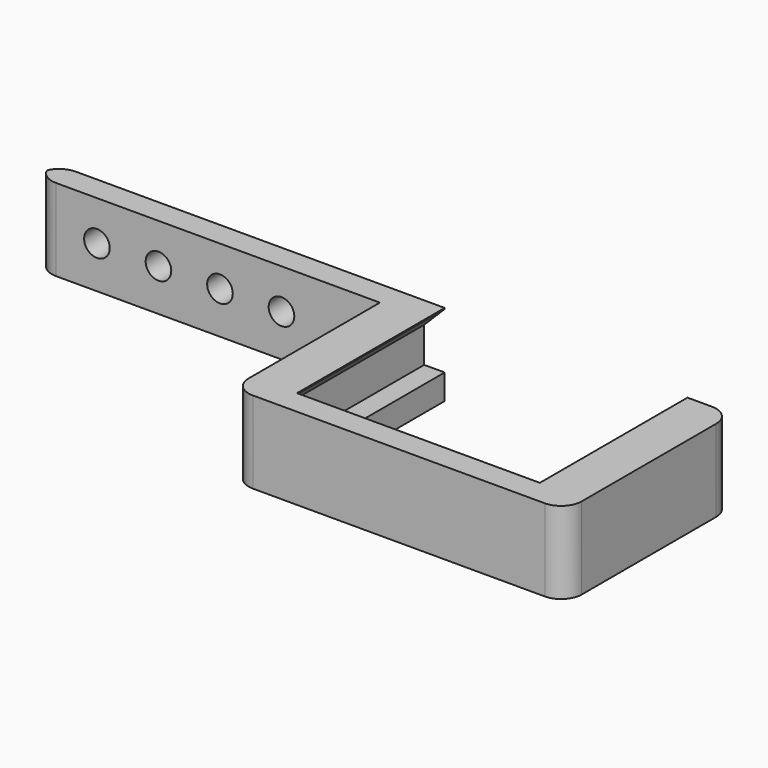
from build123d import *

# Parameters (mm, degrees)
F1_DEPTH    = 20
F3_D        = 6.2484
F4_W        = 45
F4_H        = 6.15
F4_H_2      = 5.25
F6_DEPTH    = 5
F5_W        = 45
F5_H        = 6.15
F5_H_2      = 5.25
F7_DEPTH    = 5
F8_SIZE     = 4.99999
F9_T1_DEPTH = 45
F10_R       = 5


# Not quite as in the source:
# - a fillet or chamfer that OpenCascade refuses, or shapes differently, is made with other operations: its cross-section is extruded or revolved along the edge and cut away or added
# - a fillet or chamfer is up to 0.001 mm smaller than in the source, because OpenCascade refuses the exact size


with BuildPart() as f1:
    # F0 (on Top) → F1 (new body)
    with BuildSketch(Plane.XY):
        Polygon((90, 0), (0, 0), (0, -6), (84, -6), (84, -51), (90, -51), (165.2, -51), (165.2, -45), (165.2, 0), (159.2, 0), (159.2, -45), (90, -45), align=None)
    extrude(amount=F1_DEPTH)

    # F3 (through all)
    with Locations(Plane(origin=(0, 0, 0), x_dir=(-1, 0, 0), z_dir=(0, 1, 0))):
        with Locations((-45, 10.2648036554), (-30, 10.2648036554), (-15, 10.2648036554), (-60, 10.2648036554)):
            Hole(F3_D / 2)

    # F4 (on face) → F6 (join)
    with BuildSketch(Plane(origin=(159.2, 0, 0), x_dir=(0, -1, 0), z_dir=(-1, 0, 0))):
        with Locations((22.5, 3.075)):
            Rectangle(F4_W, F4_H)
        with Locations((22.5, 17.375)):
            Rectangle(F4_W, F4_H_2)
    extrude(amount=F6_DEPTH)

    # F5 (on face) → F7 (join)
    with BuildSketch(Plane.YZ.offset(90)):
        with Locations((-22.5, 3.075)):
            Rectangle(F5_W, F5_H)
        with Locations((-22.5, 17.375)):
            Rectangle(F5_W, F5_H_2)
    extrude(amount=F7_DEPTH)

    # F8 (size 5 in the source; OpenCascade refuses exactly that, so slightly less here)
    f8_edges = [f1.edges().sort_by_distance(p)[0] for p in [
        (154.2, -22.5, 14.75),
        (95, -22.5, 14.75),
    ]]
    chamfer(f8_edges, length=F8_SIZE)

    # F9: fillet of radius 5 on 4 edges, made by hand

    # F9_s2 → F9_t1 (cut)
    with BuildSketch(Plane.XY.offset(-12.5)):
        with BuildLine():
            ThreePointArc((160.2, -51), (163.7355339059, -49.5355339059), (165.2, -46))
            Line((165.2, -46), (165.2, -51))
            Line((165.2, -51), (160.2, -51))
        make_face()
        with BuildLine():
            ThreePointArc((84, -46), (85.4644660941, -49.5355339059), (89, -51))
            Line((89, -51), (84, -51))
            Line((84, -51), (84, -46))
        make_face()
        with BuildLine():
            ThreePointArc((5, 0), (1.4644660941, -1.4644660941), (0, -5))
            Line((0, -5), (0, 0))
            Line((0, 0), (5, 0))
        make_face()
        with BuildLine():
            ThreePointArc((0, -1), (1.4644660941, -4.5355339059), (5, -6))
            Line((5, -6), (0, -6))
            Line((0, -6), (0, -1))
        make_face()
    extrude(amount=F9_T1_DEPTH, mode=Mode.SUBTRACT)

    # F10
    f10_edges = [f1.edges().sort_by_distance(p)[0] for p in [
        (165.2, 0, 10),
    ]]
    fillet(f10_edges, radius=F10_R)


solid = f1.part
